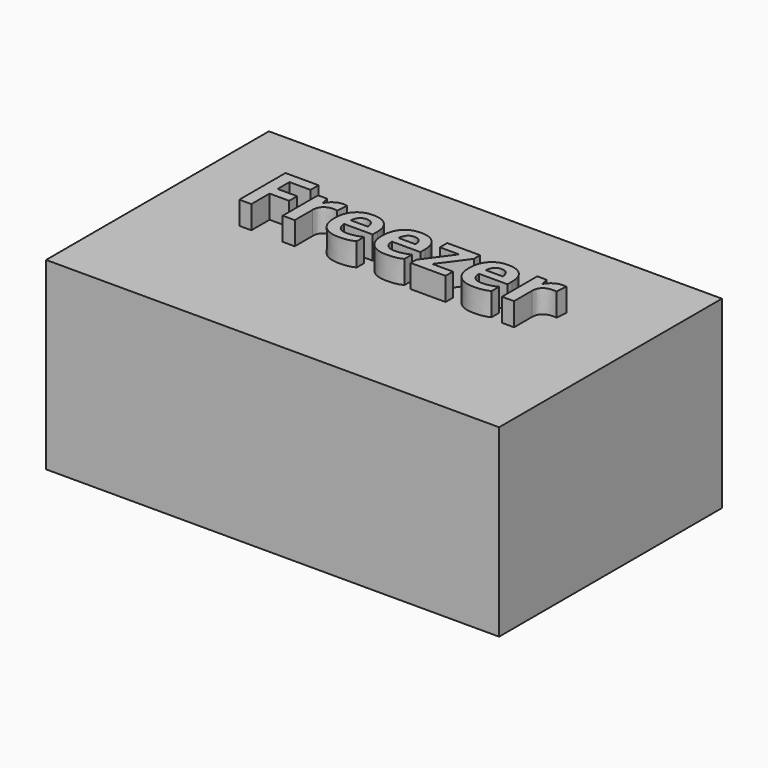
from build123d import *

# Parameters (mm, degrees)
F0_W         = 62.4053739011
F0_H         = 38.3659489453
F1_DEPTH     = 25.4
F2_TEXT_SIZE = 11.1293629743
F3_DEPTH     = 3.175


# Not quite as in the source:
# - Text() gives the source's letters only with a copy of the font that has no kerning and outlines rounded to 1/6400 em; it was checked with that copy


with BuildPart() as f1:
    # F0 (on Top) → F1 (new body)
    with BuildSketch(Plane.XY):
        Rectangle(F0_W, F0_H)
    extrude(amount=F1_DEPTH)

    # F2 (on face) → F3 (join)
    with BuildSketch(Plane.XY.offset(25.4)):
        with Locations((-20.9292887621, 0)):
            Text('Freezer', F2_TEXT_SIZE, font='Open Sans', font_style=FontStyle.BOLD, text_align=(TextAlign.LEFT, TextAlign.BOTTOM))
    extrude(amount=F3_DEPTH)


solid = f1.part
